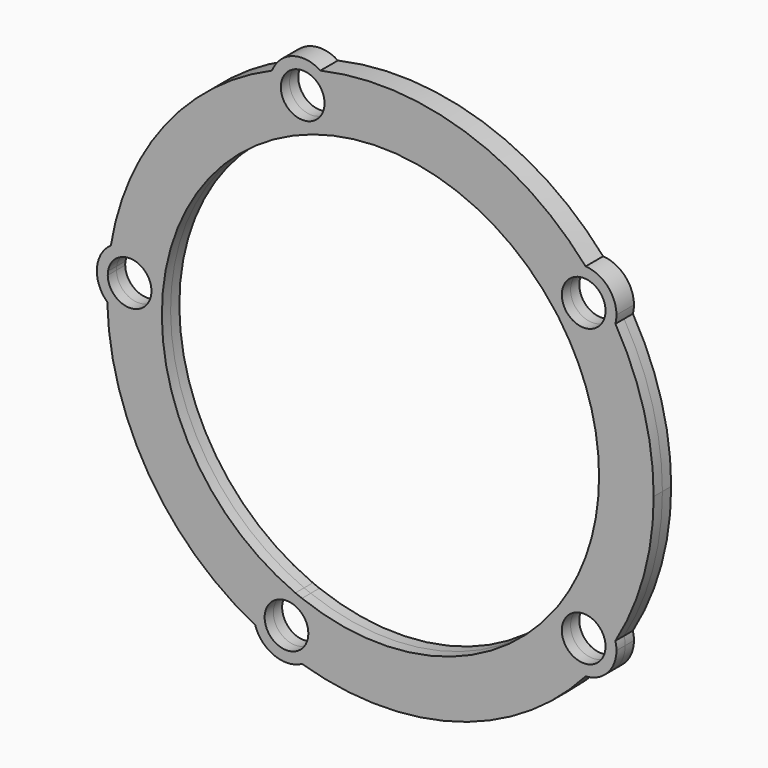
from build123d import *

# Parameters (mm, degrees)
F0_R     = 6.35
F1_DEPTH = 3.175


with BuildPart() as f1:
    # F0 (on Front) → F1 (new body, symmetric)
    with BuildSketch(Plane.XZ):
        with BuildLine():
            ThreePointArc((-17.4334869568, 77.4671706545), (-21.0250628511, 76.5704625087), (-24.5709427988, 75.5073358467))
            ThreePointArc((-24.5709427988, 75.5073358467), (-28.0634202853, 74.2801012289), (-31.4949046301, 72.8914259638))
            ThreePointArc((-31.4949046301, 72.8914259638), (-29.5170408255, 62.9143726492), (-19.6585851248, 60.4114964503))
            ThreePointArc((-19.6585851248, 60.4114964503), (-14.8988685075, 63.8720589464), (-13.081, 69.469))
            ThreePointArc((-13.081, 69.469), (-14.2395846465, 74.0218803116), (-17.4334869568, 77.4671706545))
        make_face()
        with BuildLine():
            ThreePointArc((-24.5709427988, 75.5073358467), (-18.8747057723, 74.6070875222), (-16.256, 69.469))
            ThreePointArc((-16.256, 69.469), (-26.3372942277, 64.3309124778), (-24.5709427988, 75.5073358467))
        make_face(mode=Mode.SUBTRACT)
        with BuildLine():
            ThreePointArc((-31.4949046301, 72.8914259638), (-28.0634202853, 74.2801012289), (-24.5709427988, 75.5073358467))
            ThreePointArc((-24.5709427988, 75.5073358467), (-21.0250628511, 76.5704625087), (-17.4334869568, 77.4671706545))
            ThreePointArc((-17.4334869568, 77.4671706545), (-25.5534143712, 78.5265037137), (-31.4949046301, 72.8914259638))
        make_face()
        with BuildLine():
            ThreePointArc((59.6305906851, 52.4335927744), (24.5319973939, 75.5199980174), (-17.4334869568, 77.4671706545))
            ThreePointArc((-17.4334869568, 77.4671706545), (-14.2395846465, 74.0218803116), (-13.081, 69.469))
            ThreePointArc((-13.081, 69.469), (-14.8988685075, 63.8720589464), (-19.6585851248, 60.4114964503))
            ThreePointArc((-19.6585851248, 60.4114964503), (19.192650723, 60.561134655), (50.8659607408, 38.0613046332))
            ThreePointArc((50.8659607408, 38.0613046332), (50.9228529034, 47.8852145144), (59.6305906851, 52.4335927744))
        make_face()
        with BuildLine():
            ThreePointArc((-19.6585851248, 60.4114964503), (-29.5170408255, 62.9143726492), (-31.4949046301, 72.8914259638))
            ThreePointArc((-31.4949046301, 72.8914259638), (-62.5829136435, 48.8719542947), (-78.3514836066, 12.8892984033))
            ThreePointArc((-78.3514836066, 12.8892984033), (-68.4945244609, 13.5260066408), (-63.373, 5.08))
            ThreePointArc((-63.373, 5.08), (-69.0923257109, -3.6516933183), (-79.3819172084, -1.8974237821))
            ThreePointArc((-79.3819172084, -1.8974237821), (-67.3022929991, -42.1365678923), (-36.3814305576, -70.5796040459))
            ThreePointArc((-36.3814305576, -70.5796040459), (-34.1498428756, -61.0672736312), (-24.7158919074, -58.5246406199))
            ThreePointArc((-24.7158919074, -58.5246406199), (-63.4722358852, 2.6989153756), (-19.6585851248, 60.4114964503))
        make_face()
        with BuildLine():
            ThreePointArc((68.58, 42.926), (65.9907092743, 49.4545191171), (59.6305906851, 52.4335927744))
            ThreePointArc((59.6305906851, 52.4335927744), (64.2293016822, 46.6871053087), (68.276185728, 40.5395049195))
            ThreePointArc((68.276185728, 40.5395049195), (68.5037411611, 41.7231220052), (68.58, 42.926))
        make_face()
        with BuildLine():
            ThreePointArc((68.276185728, 40.5395049195), (64.2293016822, 46.6871053087), (59.6305906851, 52.4335927744))
            ThreePointArc((59.6305906851, 52.4335927744), (50.9228529034, 47.8852145144), (50.8659607408, 38.0613046332))
            ThreePointArc((50.8659607408, 38.0613046332), (51.3882284212, 37.3531638847), (51.9006383071, 36.6378576855))
            ThreePointArc((51.9006383071, 36.6378576855), (61.2626352015, 33.6603660866), (68.276185728, 40.5395049195))
        make_face()
        with Locations((59.055, 42.926)):
            Circle(F0_R, mode=Mode.SUBTRACT)
        with BuildLine():
            ThreePointArc((-63.373, 5.08), (-68.4945244609, 13.5260066408), (-78.3514836066, 12.8892984033))
            ThreePointArc((-78.3514836066, 12.8892984033), (-78.8370586265, 9.4766652265), (-79.1740663586, 6.0461734122))
            ThreePointArc((-79.1740663586, 6.0461734122), (-72.4135009686, 11.4114896106), (-66.548, 5.08))
            ThreePointArc((-66.548, 5.08), (-72.8548244643, -1.2698532167), (-79.2474128734, 4.9936509246))
            ThreePointArc((-79.2474128734, 4.9936509246), (-79.3894691896, 1.5495736457), (-79.3819172084, -1.8974237821))
            ThreePointArc((-79.3819172084, -1.8974237821), (-69.0923257109, -3.6516933183), (-63.373, 5.08))
        make_face()
        with BuildLine():
            ThreePointArc((-79.1740663586, 6.0461734122), (-78.8370586265, 9.4766652265), (-78.3514836066, 12.8892984033))
            ThreePointArc((-78.3514836066, 12.8892984033), (-82.3999562618, 5.7421572308), (-79.3819172084, -1.8974237821))
            ThreePointArc((-79.3819172084, -1.8974237821), (-79.3894691896, 1.5495736457), (-79.2474128734, 4.9936509246))
            ThreePointArc((-79.2474128734, 4.9936509246), (-79.2326375079, 5.5214381539), (-79.1740663586, 6.0461734122))
        make_face()
        with BuildLine():
            ThreePointArc((79.4045905265, 0), (76.5719647362, 21.0195911739), (68.276185728, 40.5395049195))
            ThreePointArc((68.276185728, 40.5395049195), (61.2626352015, 33.6603660866), (51.9006383071, 36.6378576855))
            ThreePointArc((51.9006383071, 36.6378576855), (60.5526018111, 19.2195547913), (63.5295905265, 0))
            ThreePointArc((63.5295905265, 0), (60.5526018111, -19.2195547913), (51.9006383071, -36.6378576855))
            ThreePointArc((51.9006383071, -36.6378576855), (61.2626352015, -33.6603660866), (68.276185728, -40.5395049195))
            ThreePointArc((68.276185728, -40.5395049195), (76.5719647362, -21.0195911739), (79.4045905265, 0))
        make_face()
        with BuildLine():
            ThreePointArc((-22.8093313363, -59.2937035145), (-23.7657227015, -58.9168846507), (-24.7158919074, -58.5246406199))
            ThreePointArc((-24.7158919074, -58.5246406199), (-34.1498428756, -61.0672736312), (-36.3814305576, -70.5796040459))
            ThreePointArc((-36.3814305576, -70.5796040459), (-29.7043860041, -73.6392453031), (-22.7732002069, -76.0688526864))
            ThreePointArc((-22.7732002069, -76.0688526864), (-19.1229764719, -72.5674860284), (-17.78, -67.691))
            ThreePointArc((-17.78, -67.691), (-19.1334986379, -62.7969024847), (-22.8093313363, -59.2937035145))
        make_face()
        with Locations((-27.305, -67.691)):
            Circle(F0_R, mode=Mode.SUBTRACT)
        with BuildLine():
            ThreePointArc((-22.7732002069, -76.0688526864), (-29.7043860041, -73.6392453031), (-36.3814305576, -70.5796040459))
            ThreePointArc((-36.3814305576, -70.5796040459), (-30.8681979815, -76.5244163914), (-22.7732002069, -76.0688526864))
        make_face()
        with BuildLine():
            ThreePointArc((50.8659607408, -38.0613046332), (17.5925354611, -61.0451600745), (-22.8093313363, -59.2937035145))
            ThreePointArc((-22.8093313363, -59.2937035145), (-19.1334986379, -62.7969024847), (-17.78, -67.691))
            ThreePointArc((-17.78, -67.691), (-19.1229764719, -72.5674860284), (-22.7732002069, -76.0688526864))
            ThreePointArc((-22.7732002069, -76.0688526864), (21.892308832, -76.3270319788), (59.6305906851, -52.4335927744))
            ThreePointArc((59.6305906851, -52.4335927744), (50.9228529034, -47.8852145144), (50.8659607408, -38.0613046332))
        make_face()
        with BuildLine():
            ThreePointArc((68.58, -42.926), (68.5037411611, -41.7231220052), (68.276185728, -40.5395049195))
            ThreePointArc((68.276185728, -40.5395049195), (64.2293016822, -46.6871053087), (59.6305906851, -52.4335927744))
            ThreePointArc((59.6305906851, -52.4335927744), (65.9907092743, -49.4545191171), (68.58, -42.926))
        make_face()
        with BuildLine():
            ThreePointArc((59.6305906851, -52.4335927744), (64.2293016822, -46.6871053087), (68.276185728, -40.5395049195))
            ThreePointArc((68.276185728, -40.5395049195), (61.2626352015, -33.6603660866), (51.9006383071, -36.6378576855))
            ThreePointArc((51.9006383071, -36.6378576855), (51.3882284212, -37.3531638847), (50.8659607408, -38.0613046332))
            ThreePointArc((50.8659607408, -38.0613046332), (50.9228529034, -47.8852145144), (59.6305906851, -52.4335927744))
        make_face()
        with Locations((59.055, -42.926)):
            Circle(F0_R, mode=Mode.SUBTRACT)
    extrude(amount=F1_DEPTH, both=True)


solid = f1.part
